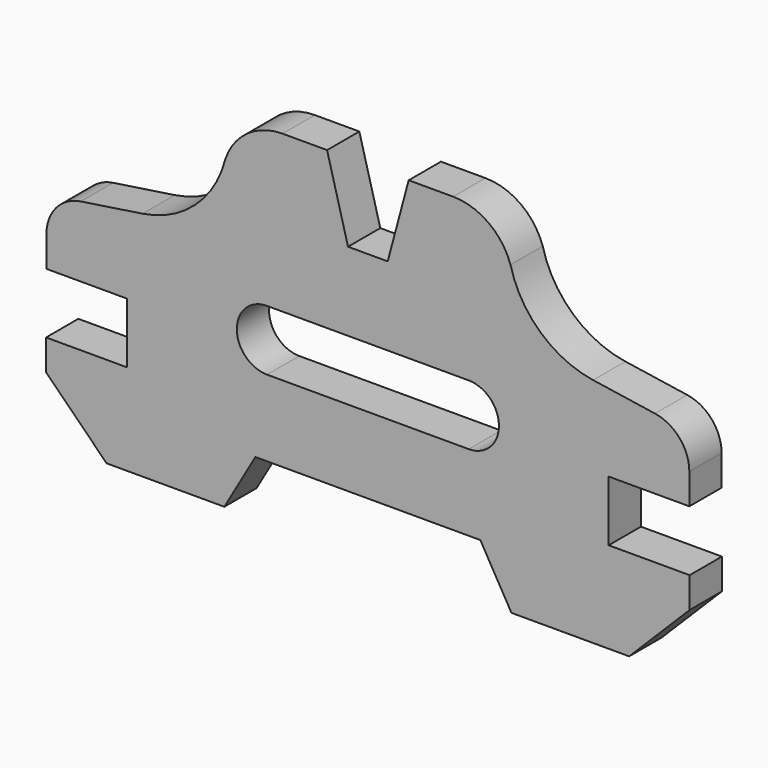
from build123d import *

# Parameters (mm, degrees)
F1_DEPTH = 6.35
F2_SIZE2 = 19.05
F2_SIZE  = 19.05
F3_SIZE2 = 19.05
F3_SIZE  = 19.05


# Not quite as in the source:
# - ends of sketch curves that miss each other by under 0.0002 mm in the source are joined


with BuildPart() as f1:
    # F0 (on Front) → F1 (new body, symmetric)
    with BuildSketch(Plane.XZ):
        with BuildLine():
            Line((101.3459994669, -21.8439942511), (75.8431146328, -21.8439942511))
            Line((75.8431146328, -21.8439942511), (75.8431146328, -2.7939942511))
            Line((75.8431146328, -2.7939942511), (101.2431146328, -2.7939942511))
            Line((101.2431146328, -2.7939942511), (101.2431146328, 6.8580057489))
            ThreePointArc((101.2431146328, 6.8580057489), (98.1684202272, 15.1431425742), (90.4331158589, 19.4165843056))
            Line((90.4331158589, 19.4165843056), (70.9499079155, 22.3487064989))
            ThreePointArc((70.9499079155, 22.3487064989), (54.3920764202, 30.184519391), (44.9188305794, 45.8631469058))
            ThreePointArc((44.9188305794, 45.8631469058), (37.9835870307, 55.281692466), (26.8519516779, 58.8724163371))
            Line((26.8519516779, 58.8724163371), (12.8488468359, 58.8724155428))
            Line((12.8488468359, 58.8724155428), (6.2471146328, 34.2344155428))
            Line((6.2471146328, 34.2344155428), (-6.2471205082, 34.2344155428))
            Line((-6.2471205082, 34.2344155428), (-12.848854109, 58.8724148139))
            Line((-12.848854109, 58.8724148139), (-26.8519589509, 58.8724148139))
            ThreePointArc((-26.8519589509, 58.8724148139), (-37.9835941001, 55.2816903113), (-44.9188371145, 45.8631443577))
            ThreePointArc((-44.9188371145, 45.8631443577), (-54.3920820431, 30.1845162803), (-70.9499131167, 22.3487024742))
            Line((-70.9499131167, 22.3487024742), (-90.4331208938, 19.4165791758))
            ThreePointArc((-90.4331208938, 19.4165791758), (-98.1684250197, 15.1431370056), (-101.2431189553, 6.8580000058))
            Line((-101.2431189553, 6.8580000058), (-101.2431189553, -2.7939999942))
            Line((-101.2431189553, -2.7939999942), (-75.8431173272, -2.7939999942))
            Line((-75.8431173272, -2.7939999942), (-75.8431173272, -21.8439985533))
            Line((-75.8431173272, -21.8439985533), (-101.3460021612, -21.844))
            Line((-101.3460021612, -21.844), (-101.3460005331, -50.546))
            Line((-101.3460005331, -50.546), (-45.2120005331, -50.5459968158))
            Line((-45.2120005331, -50.5459968158), (-35.4220414842, -33.5504287171))
            Line((-35.4220414842, -33.5504287171), (-1.0151e-06, -33.5504287171))
            Line((-1.0151e-06, -33.5504287171), (35.4220394539, -33.5504267077))
            Line((35.4220394539, -33.5504267077), (45.2119994669, -50.5459942511))
            Line((45.2119994669, -50.5459942511), (101.3459994669, -50.5459942511))
            Line((101.3459994669, -50.5459942511), (101.3459994669, -21.8439942511))
        make_face()
        with BuildLine():
            Line((-31.7500042241, 9.525), (31.7499957759, 9.525))
            ThreePointArc((31.7499957759, 9.525), (41.2750042241, 4.2241e-06), (31.7500042241, -9.525))
            Line((31.7500042241, -9.525), (-31.7499957759, -9.525))
            ThreePointArc((-31.7499957759, -9.525), (-41.2750042241, -4.2241e-06), (-31.7500042241, 9.525))
        make_face(mode=Mode.SUBTRACT)
    extrude(amount=F1_DEPTH, both=True)

    # F2
    f2_edges = [f1.edges().sort_by_distance(p)[0] for p in [
        (101.345999, 0, -50.545994),
    ]]
    chamfer(f2_edges, length=F2_SIZE, length2=F2_SIZE2)

    # F3
    f3_edges = [f1.edges().sort_by_distance(p)[0] for p in [
        (-101.346001, 0, -50.546),
    ]]
    chamfer(f3_edges, length=F3_SIZE, length2=F3_SIZE2)


solid = f1.part
